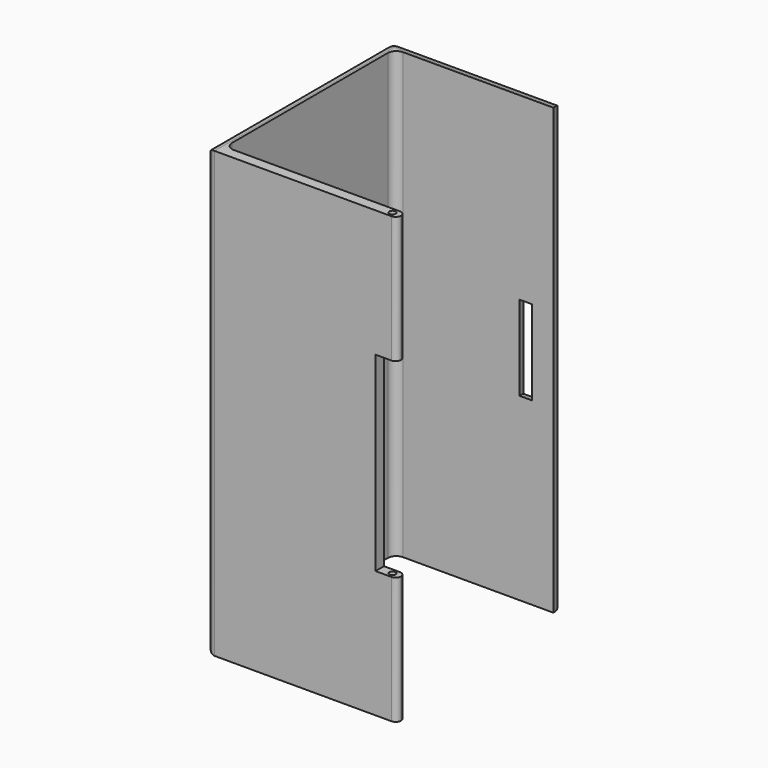
from build123d import *

# Parameters (mm, degrees)
F0_W      = 127
F0_H      = 266.7
F1_DEPTH  = 139.7
F2_T      = -6.35
F3_R      = 5.08
F4_DEPTH  = 25.4
F5_W      = 7.62
F5_H      = 50.8
F6_DEPTH  = 25.4
F7_R      = 1.905
F8_DEPTH  = 266.701
F9_R      = 5.08
F11_W     = 6.35
F11_H     = 76.2
F12_DEPTH = 12.7
F13_DEPTH = 266.701
F14_R     = 3.17499


# Not quite as in the source:
# - a fillet or chamfer is up to 0.001 mm smaller than in the source, because OpenCascade refuses the exact size


with BuildPart() as f1:
    # F0 (on Front) → F1 (new body)
    with BuildSketch(Plane.XZ):
        with Locations((-63.5, -133.35)):
            Rectangle(F0_W, F0_H)
    extrude(amount=F1_DEPTH)

    # F2
    f2_openings = [f1.faces().sort_by_distance(p)[0] for p in [
        (-63.5, -69.85, -266.7),
        (-63.5, -69.85, 0),
    ]]
    offset(amount=F2_T, openings=f2_openings)

    # F3
    f3_edges = [f1.edges().sort_by_distance(p)[0] for p in [
        (-6.35, -133.35, -133.35),
        (-120.65, -133.35, -133.35),
        (-6.35, -6.35, -133.35),
        (-120.65, -6.35, -133.35),
    ]]
    fillet(f3_edges, radius=F3_R)

    # F4 (cut): a face of the model
    f4_faces = [f1.faces().sort_by_distance(p)[0] for p in [
        (0, -69.85, -133.35),
    ]]
    extrude(f4_faces, amount=-F4_DEPTH, mode=Mode.SUBTRACT)

    # F5 (on face) → F6 (cut)
    with BuildSketch(Plane(origin=(0, 0, 0), x_dir=(-1, 0, 0), z_dir=(0, 1, 0))):
        with Locations((41.91, -133.35)):
            Rectangle(F5_W, F5_H)
    extrude(amount=-F6_DEPTH, mode=Mode.SUBTRACT)

    # F7 (on face) → F8 (cut, through all)
    with BuildSketch(Plane(origin=(0, 0, -266.7), x_dir=(1, 0, 0), z_dir=(0, 0, -1))):
        with Locations((-17.78, 136.525)):
            Circle(F7_R)
    extrude(amount=-F8_DEPTH, mode=Mode.SUBTRACT)

    # F9
    f9_edges = [f1.edges().sort_by_distance(p)[0] for p in [
        (-127, 0, -133.35),
        (-127, -69.85, -266.7),
        (-127, -69.85, 0),
        (-127, -139.7, -133.35),
        (-25.4, 0, -133.35),
        (-76.2, 0, -266.7),
        (-76.2, 0, 0),
        (-45.72, 0, -133.35),
        (-41.91, 0, -158.75),
        (-38.1, 0, -133.35),
        (-41.91, 0, -107.95),
    ]]
    fillet(f9_edges, radius=F9_R)

    # F11 (on offset) → F12 (join)
    with BuildSketch(Plane.YZ.offset(-25.4)):
        with Locations((-136.525, -38.1)):
            Rectangle(F11_W, F11_H)
        with Locations((-136.525, -228.6)):
            Rectangle(F11_W, F11_H)
    extrude(amount=F12_DEPTH)

    # F7 (on face) → F13 (cut, through all)
    with BuildSketch(Plane(origin=(0, 0, -266.7), x_dir=(1, 0, 0), z_dir=(0, 0, -1))):
        with Locations((-17.78, 136.525)):
            Circle(F7_R)
    extrude(amount=-F13_DEPTH, mode=Mode.SUBTRACT)

    # F14 (radius 3.175 in the source; OpenCascade refuses exactly that, so slightly less here)
    f14_edges = [f1.edges().sort_by_distance(p)[0] for p in [
        (-12.7, -133.35, -228.6),
        (-12.7, -133.35, -38.1),
        (-12.7, -139.7, -38.1),
        (-12.7, -139.7, -228.6),
    ]]
    fillet(f14_edges, radius=F14_R)


solid = f1.part
